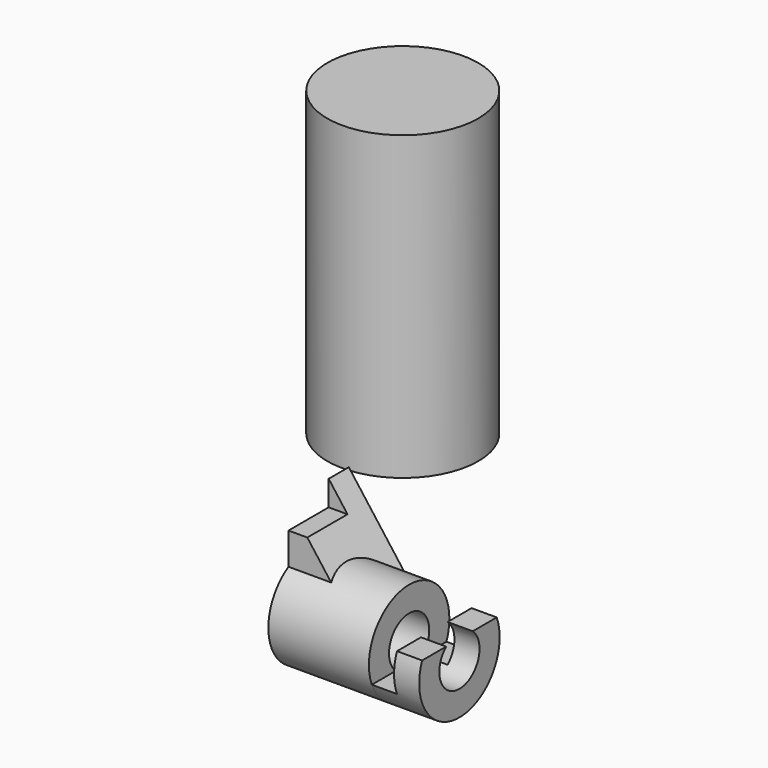
from build123d import *

# Parameters (mm, degrees)
F0_R      = 25.4
F0_R_2    = 12.7
F1_DEPTH  = 50.8
F3_DEPTH  = 12.7
F5_DEPTH  = 12.7
F8_DEPTH  = 38.1
F9_DEPTH  = 50.801
F10_W     = 25.4
F10_H     = 12.7
F11_DEPTH = 25.4
F12_R     = 38.1
F13_DEPTH = 152.4


with BuildPart() as f1:
    # F0 (on Right) → F1 (new body)
    with BuildSketch(Plane.YZ):
        Circle(F0_R)
        Circle(F0_R_2, mode=Mode.SUBTRACT)
    extrude(amount=F1_DEPTH)

    # F2 (on face) → F3 (join)
    with BuildSketch(Plane.YZ.offset(50.8)):
        with BuildLine():
            Line((-8.4002604126, -9.525), (-23.5464301965, -9.525))
            ThreePointArc((-23.5464301965, -9.525), (0, -25.4), (23.5464301965, -9.525))
            Line((23.5464301965, -9.525), (8.4002604126, -9.525))
            ThreePointArc((8.4002604126, -9.525), (0, -12.7), (-8.4002604126, -9.525))
        make_face()
    extrude(amount=F3_DEPTH)

    # F4 (on face) → F5 (join)
    with BuildSketch(Plane.YZ.offset(63.5)):
        with BuildLine():
            Line((-8.4002604126, 9.525), (-23.5464301965, 9.525))
            ThreePointArc((-23.5464301965, 9.525), (-25.4, 0), (-23.5464301965, -9.525))
            Line((-23.5464301965, -9.525), (-8.4002604126, -9.525))
            ThreePointArc((-8.4002604126, -9.525), (-12.7, 0), (-8.4002604126, 9.525))
        make_face()
        with BuildLine():
            ThreePointArc((23.5464301965, -9.525), (25.4, 0), (23.5464301965, 9.525))
            Line((23.5464301965, 9.525), (8.4002604126, 9.525))
            ThreePointArc((8.4002604126, 9.525), (12.7, 0), (8.4002604126, -9.525))
            Line((8.4002604126, -9.525), (23.5464301965, -9.525))
        make_face()
        with BuildLine():
            Line((-8.4002604126, -9.525), (-23.5464301965, -9.525))
            ThreePointArc((-23.5464301965, -9.525), (0, -25.4), (23.5464301965, -9.525))
            Line((23.5464301965, -9.525), (8.4002604126, -9.525))
            ThreePointArc((8.4002604126, -9.525), (0, -12.7), (-8.4002604126, -9.525))
        make_face()
    extrude(amount=F5_DEPTH)

    # F7 (on offset) → F8 (join)
    with BuildSketch(Plane.XZ.offset(-25.4)):
        Polygon((0, 50.8), (0, 0), (38.1, 0), align=None)
    extrude(amount=F8_DEPTH)

    # F2 (on face) → F9 (cut, through all)
    with BuildSketch(Plane.YZ.offset(50.8)):
        with BuildLine():
            ThreePointArc((8.4002604126, 9.525), (0, 12.7), (-8.4002604126, 9.525))
            Line((-8.4002604126, 9.525), (8.4002604126, 9.525))
        make_face()
        with BuildLine():
            Line((8.4002604126, 9.525), (-8.4002604126, 9.525))
            ThreePointArc((-8.4002604126, 9.525), (-12.7, 0), (-8.4002604126, -9.525))
            Line((-8.4002604126, -9.525), (8.4002604126, -9.525))
            ThreePointArc((8.4002604126, -9.525), (11.5752604126, -5.2252604126), (12.7, 0))
            ThreePointArc((12.7, 0), (11.5752604126, 5.2252604126), (8.4002604126, 9.525))
        make_face()
    extrude(amount=-F9_DEPTH, mode=Mode.SUBTRACT)

    # F10 (on face) → F11 (cut)
    with BuildSketch(Plane(origin=(0, 0, 0), x_dir=(0, -1, 0), z_dir=(-1, 0, 0))):
        with Locations((0, 44.45)):
            Rectangle(F10_W, F10_H)
    extrude(amount=-F11_DEPTH, mode=Mode.SUBTRACT)


with BuildPart() as f13:
    # F12 (on Top) → F13 (new body)
    with BuildSketch(Plane.XY):
        with Locations((-62.3511075974, 137.4269872904)):
            Circle(F12_R)
    extrude(amount=F13_DEPTH)


solid = Compound([f1.part, f13.part])
